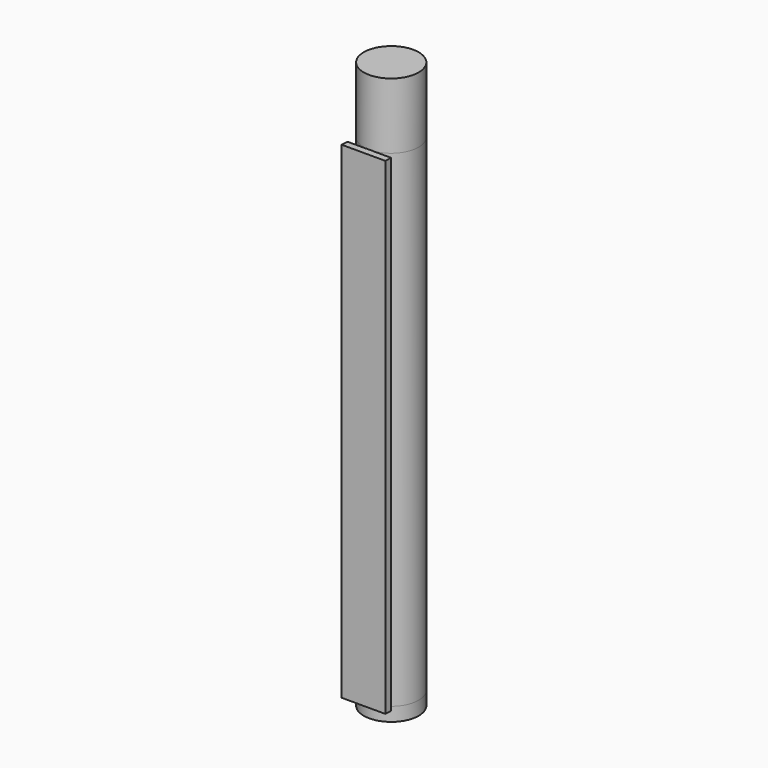
from build123d import *

# Parameters (mm, degrees)
F1_DEPTH = 112.7125
F2_R     = 6.35
F3_DEPTH = 15.24
F4_R     = 6.35
F5_DEPTH = 3.175


with BuildPart() as f1:
    # F0 (on Top) → F1 (new body)
    with BuildSketch(Plane.XY):
        with BuildLine():
            Line((0.762, -6.35), (0.762, -6.304114))
            ThreePointArc((0.762, -6.304114), (0, 6.35), (-0.762, -6.304114))
            Line((-0.762, -6.304114), (-0.762, -6.35))
            Line((-0.762, -6.35), (-5.0419, -6.35))
            Line((-5.0419, -6.35), (-5.11427, -7.93585))
            Line((-5.11427, -7.93585), (4.96953, -7.93585))
            Line((4.96953, -7.93585), (5.0419, -6.35))
            Line((5.0419, -6.35), (0.762, -6.35))
        make_face()
    extrude(amount=F1_DEPTH)

    # F2 (on face) → F3 (join)
    with BuildSketch(Plane.XY.offset(112.7125)):
        Circle(F2_R)
    extrude(amount=F3_DEPTH)

    # F4 (on face) → F5 (join)
    with BuildSketch(Plane(origin=(0, 0, 0), x_dir=(1, 0, 0), z_dir=(0, 0, -1))):
        Circle(F4_R)
    extrude(amount=F5_DEPTH)


solid = f1.part
